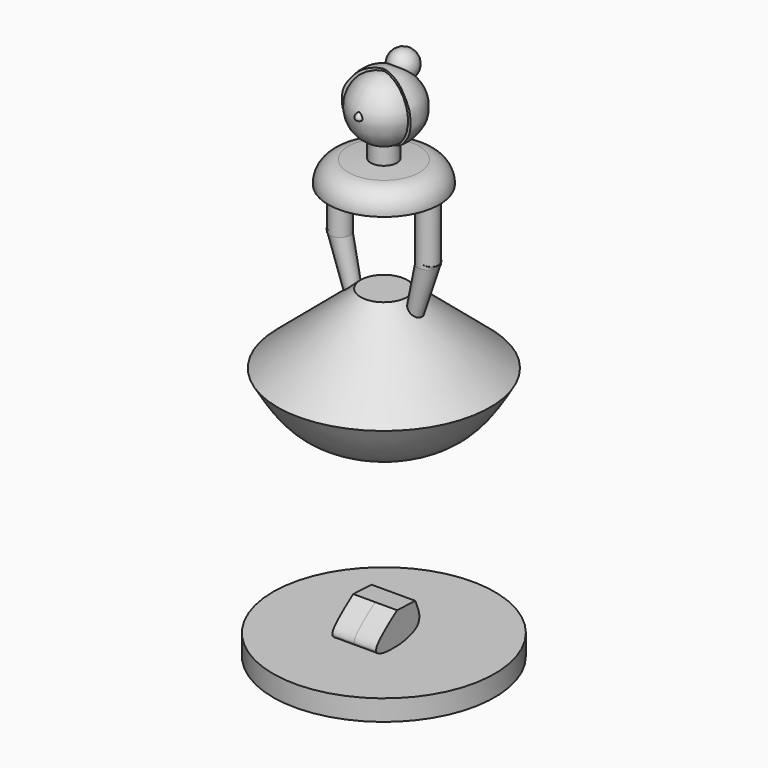
from build123d import *

# Parameters (mm, degrees)
F10_W          = 1.942879986
F10_H          = 2.8718784451
F21_DEPTH      = 3.25
F21_DEPTH_BACK = 3.25
F23_ANGLE_BACK = 17.9542385382
F23_ANGLE      = 212.9542385382
F28_W          = 16.4624936879
F28_H          = 3.0818809102


# Not quite as in the source:
# - the program builds the solid bodies; features that only make, move or delete a surface that nothing else refers to are left out


with BuildPart() as f3:
    # F2 (on Front) → F3 (revolve)
    with BuildSketch(Plane.XZ):
        with BuildLine():
            Line((0, 27.5518217697), (-5.2735735662, 27.2742658854))
            ThreePointArc((-5.2735735662, 27.2742658854), (-7.4179399127, 26.2642214143), (-8.2426649549, 24.0419870734))
            Line((-8.2426649549, 24.0419870734), (-5.1087746397, 24.1430792958))
            Line((-5.1087746397, 24.1430792958), (0, 24.1430792958))
            Line((0, 24.1430792958), (0, 27.5518217697))
        make_face()
    revolve(axis=Axis((0, 0, 25.8474505327), (0, 0, 1)))

    # F10 (on Front) → F11 (revolve)
    with BuildSketch(Plane.XZ):
        with Locations((-0.971439993, 28.5847540945)):
            Rectangle(F10_W, F10_H)
    revolve(axis=Axis((0, 0, 28.5847540945), (0, 0, -1)))

    # F12 (on Front) → F13 (revolve)
    with BuildSketch(Plane.XZ):
        with BuildLine():
            Line((0, 29.5958910137), (0, 38.8363413513))
            ThreePointArc((0, 38.8363413513), (-4.7332113408, 34.2161161825), (0, 29.5958910137))
        make_face()
    revolve(axis=Axis((0, 0, 34.2161161825), (0, 0, -1)))

    # F14 (on Right) → F15 (revolve)
    with BuildSketch(Plane.YZ):
        with BuildLine():
            Line((-4.5526074246, 34.156948328), (-4.5526074246, 35.377189517))
            add(Edge.make_bspline(
                [(-4.5526074246, 35.377189517), (-5.0519458341, 35.1065115565), (-5.2583922065, 34.4336617904), (-4.9682680601, 34.3008922752), (-4.5526074246, 34.156948328)],
                knots=[0, 0, 0, 0, 0.5499379452, 1, 1, 1, 1], degree=3))
        make_face()
    revolve(axis=Axis((0, -4.5526074246, 34.7670689225), (0, 0, -1)))


with BuildPart() as f5:
    # F4 (on Front) → F5 (revolve)
    with BuildSketch(Plane.XZ):
        Polygon((-6.531172432, 24.504929781), (-8.0504994839, 24.0633841604), (-8.0504994839, 15.7383214682), (-6.531172432, 15.7383214682), align=None)
    revolve(axis=Axis((-6.531172432, 0, 20.1216256246), (0, 0, 1)))


with BuildPart() as f7:
    # F6 (on Front) → F7 (revolve)
    with BuildSketch(Plane.XZ):
        Polygon((-6.5701799467, 16.0351097584), (-8.1108621801, 16.0351097584), (-5.66249853, 8.5390601307), (-4.6435656187, 8.8718645311), align=None)
    revolve(axis=Axis((-5.6068727827, 0, 12.4534871448), (0.2597281384, 0, -0.9656817768)))


with BuildPart() as f8_1:
    # F8: instance of F5
    add(f5.part.mirror(Plane.YZ))


with BuildPart() as f9_1:
    # F9: instance of F7
    add(f7.part.mirror(Plane.YZ))


with BuildPart() as f17:
    # F16 (on Front) → F17 (revolve)
    with BuildSketch(Plane.XZ):
        with BuildLine():
            Line((0, 10.3970682248), (-3.4505850635, 10.3970682248))
            Line((-3.4505850635, 10.3970682248), (-15.7853383571, 0))
            add(Edge.make_bspline(
                [(-15.7853383571, 0), (-14.3352225564, -2.4834041203), (-11.2219147866, -7.8151171734), (-3.9075054059, -9.4796002192), (0, -10.3688007221)],
                knots=[0, 0, 0, 0, 0.4657797776, 1, 1, 1, 1], degree=3))
            Line((0, -10.3688007221), (0, 10.3970682248))
        make_face()
    revolve(axis=Axis((0, 0, 0.0141337514), (0, 0, -1)))


with BuildPart() as f21:
    # F20 (on Right) → F21 (new body, two sides)
    with BuildSketch(Plane.YZ) as f21_sk:
        with BuildLine():
            add(Edge.make_bspline(
                [(1.7842429224, -30.088827014), (2.3918488427, -31.4575260785), (3.8684294428, -34.7836860432), (-8.7195195464, -35.0121502759), (-3.8741257884, -31.5403003046), (-1.6220395919, -29.9266222864)],
                knots=[0, 0, 0, 0, 0.2723203311, 0.6617824227, 1, 1, 1, 1], degree=3))
            Line((1.7842429224, -30.088827014), (-1.6220395919, -29.9266222864))
        make_face()
    extrude(amount=F21_DEPTH)
    extrude(f21_sk.sketch, amount=-F21_DEPTH_BACK)


with BuildPart() as f23:
    # F22 (on Front) → F23 (revolve)
    with BuildSketch(Plane.XZ, mode=Mode.PRIVATE) as f23_sk:
        with BuildLine():
            add(Edge.make_bspline(
                [(0, 38.290578872), (-0.935706285, 37.9555052265), (-2.7181885983, 37.3172035968), (-3.6397820324, 34.9742782904), (-3.846231697, 33.6469820621), (-3.7869249568, 32.2802882233), (-3.3793785924, 31.2564321488), (-3.162242705, 30.71093373)],
                knots=[0, 0, 0, 0, 0.2468814523, 0.4702990983, 0.6403513124, 0.8083834288, 1, 1, 1, 1], degree=3))
            Line((0, 38.290578872), (0, 39.1113050282))
            add(Edge.make_bspline(
                [(0, 39.1113050282), (-0.2317898992, 39.1288173185), (-0.8118231527, 39.1726402407), (-2.5978105798, 38.7151687112), (-3.8800893093, 37.5593760472), (-5.0396533312, 35.9428061332), (-5.2316241134, 34.5954121219), (-5.1936265627, 32.6682793647), (-4.2404569787, 31.4814913618), (-3.8127490236, 30.8874199719), (-2.9843565927, 30.2518025622), (-2.3127425162, 30.0760779039), (-1.9713852089, 29.986763373)],
                knots=[0, 0, 0, 0, 0.0765207122, 0.1914861598, 0.3071878701, 0.426619659, 0.5277542423, 0.6464085829, 0.7507671921, 0.8248438509, 0.9109744219, 1, 1, 1, 1], degree=3))
            add(Edge.make_bspline(
                [(-3.162242705, 30.71093373), (-2.9723530738, 30.5703658588), (-2.5945058701, 30.2906603439), (-2.1783828374, 30.0877164567), (-1.9713852089, 29.986763373)],
                knots=[0, 0, 0, 0, 0.5025566667, 1, 1, 1, 1], degree=3))
        make_face()
    revolve(f23_sk.sketch.rotate(Axis((0, 0, 34.5475208014), (0, 0, -1)), -F23_ANGLE_BACK), axis=Axis((0, 0, 34.5475208014), (0, 0, -1)), revolution_arc=F23_ANGLE)


with BuildPart() as f27:
    # F26 (on Right) → F27 (revolve)
    with BuildSketch(Plane.YZ):
        with BuildLine():
            Line((1.9792781005, 39.6272717753), (5.1605091802, 37.0209624879))
            ThreePointArc((5.1605091802, 37.0209624879), (4.877050463, 39.9196176849), (1.9792781005, 39.6272717753))
        make_face()
    revolve(axis=Axis((0, 3.5254069662, 38.3605640382), (0, 0.7735419561, -0.6337450924)))


with BuildPart() as f29:
    # F28 (on Front) → F29 (revolve)
    with BuildSketch(Plane.XZ):
        with Locations((-8.2312468439, -36.1377930129)):
            Rectangle(F28_W, F28_H)
    revolve(axis=Axis((0, 0, -36.1377930129), (0, 0, -1)))


solid = Compound([f3.part, f5.part, f7.part, f8_1.part, f9_1.part, f17.part, f21.part, f23.part, f27.part, f29.part])
